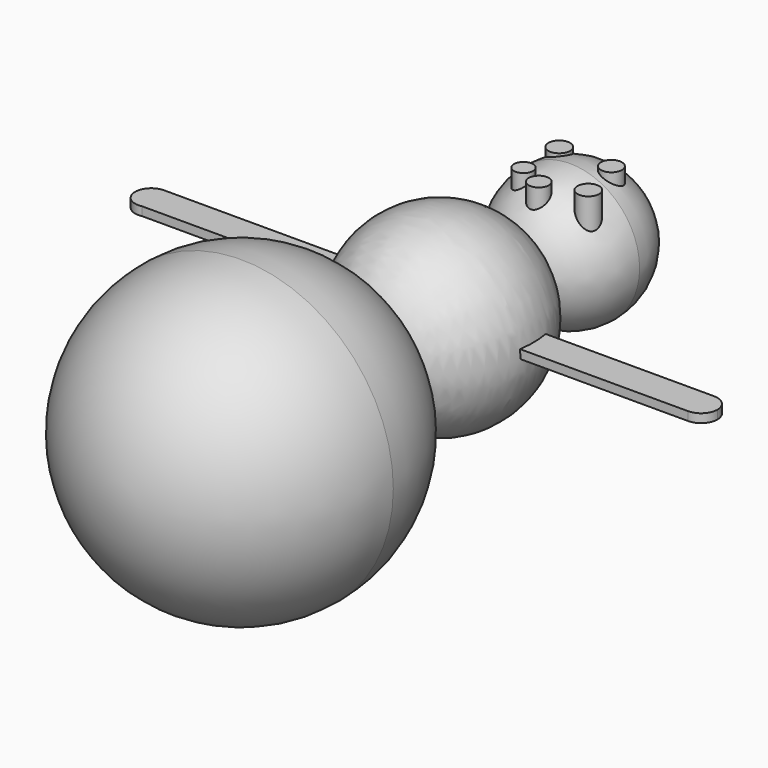
from build123d import *

# Parameters (mm, degrees)
F7_DEPTH = 1.27
F8_R     = 1.5868526343
F8_R_2   = 1.5868509173
F8_R_3   = 1.5394717584
F8_R_4   = 1.4655351759
F8_R_5   = 1.3843
F9_DEPTH = 10.16


# Not quite as in the source:
# - a feature of the source that left no trace in its solid (it failed there, or was rolled back) is left out


with BuildPart() as f1:
    # F0 (on Top) → F1 (revolve)
    with BuildSketch(Plane.XY):
        with BuildLine():
            Line((0, 27.7320817113), (0, 0))
            ThreePointArc((0, 0), (13.7653189135, 13.8660408556), (0, 27.7320817113))
        make_face()
    revolve(axis=Axis((0, 13.8660408556, 0), (0, -1, 0)))

    # F6 (on Top) → F7 (join)
    with BuildSketch(Plane.XY):
        with BuildLine():
            ThreePointArc((-42.2269459649, 12.2550480304), (-40.8876717925, 13.0777990352), (-40.3635394316, 14.5596424118))
            ThreePointArc((-40.3635394316, 14.5596424118), (-41.0538369392, 16.2261680167), (-42.7203625441, 16.9164655242))
            ThreePointArc((-42.7203625441, 16.9164655242), (-45.0640921025, 14.3115558538), (-42.2269459649, 12.2550480304))
        make_face()
        with BuildLine():
            ThreePointArc((-42.7203625441, 16.9164655242), (-41.0538369392, 16.2261680167), (-40.3635394316, 14.5596424118))
            ThreePointArc((-40.3635394316, 14.5596424118), (-40.8876717925, 13.0777990352), (-42.2269459649, 12.2550480304))
            Line((-42.2269459649, 12.2550480304), (-13.062856888, 12.2550480304))
            Line((-13.062856888, 12.2550480304), (-12.2464289889, 16.9164655242))
            Line((-12.2464289889, 16.9164655242), (-42.7203625441, 16.9164655242))
        make_face()
        with BuildLine():
            ThreePointArc((38.1019487977, 11.6428758636), (39.7795463046, 12.3377595031), (40.4744299442, 14.0153570101))
            ThreePointArc((40.4744299442, 14.0153570101), (39.7795463046, 15.692954517), (38.1019487977, 16.3878381566))
            ThreePointArc((38.1019487977, 16.3878381566), (35.7294676512, 14.0153570101), (38.1019487977, 11.6428758636))
        make_face()
        with BuildLine():
            ThreePointArc((38.1019487977, 11.6428758636), (35.7294676512, 14.0153570101), (38.1019487977, 16.3878381566))
            Line((38.1019487977, 16.3878381566), (12.7907143906, 16.3878381566))
            Line((12.7907143906, 16.3878381566), (12.2464289889, 11.6428758636))
            Line((12.2464289889, 11.6428758636), (38.1019487977, 11.6428758636))
        make_face()
    extrude(amount=F7_DEPTH)


with BuildPart() as f3:
    # F2 (on Top) → F3 (revolve)
    with BuildSketch(Plane.XY):
        with BuildLine():
            Line((0, -22.4517844617), (0, -44.7247281168))
            ThreePointArc((0, -44.7247281168), (15.7493494955, -38.2011339572), (22.272943655, -22.4517844617))
            ThreePointArc((22.272943655, -22.4517844617), (15.7493494955, -6.7024349663), (0, -0.1788408067))
            Line((0, -0.1788408067), (0, -22.4517844617))
        make_face()
    revolve(axis=Axis((0, -22.3623640584, 0), (0, 1, 0)))


with BuildPart() as f5:
    # F4 (on Top) → F5 (revolve)
    with BuildSketch(Plane.XY):
        with BuildLine():
            ThreePointArc((0, 27.5317868853), (7.1842048969, 30.5075819884), (10.16, 37.6917868853))
            ThreePointArc((10.16, 37.6917868853), (7.1842048969, 44.8759917821), (0, 47.8517868853))
            Line((0, 47.8517868853), (0, 27.5317868853))
        make_face()
    revolve(axis=Axis((0, 37.6917868853, 0), (0, -1, 0)))

    # F8 (on Top) → F9 (join)
    with BuildSketch(Plane.XY):
        with Locations((-3.5378572065, 40.1410721242)):
            Circle(F8_R)
        with Locations((5.7150004432, 33.8817872107)):
            Circle(F8_R_2)
        with Locations((4.0821437724, 40.1410721242)):
            Circle(F8_R_3)
        with Locations((0, 31.9767855108)):
            Circle(F8_R_4)
        with Locations((-3.5378572065, 33.6096435785)):
            Circle(F8_R_5)
    extrude(amount=F9_DEPTH)


solid = Compound([f1.part, f3.part, f5.part])
